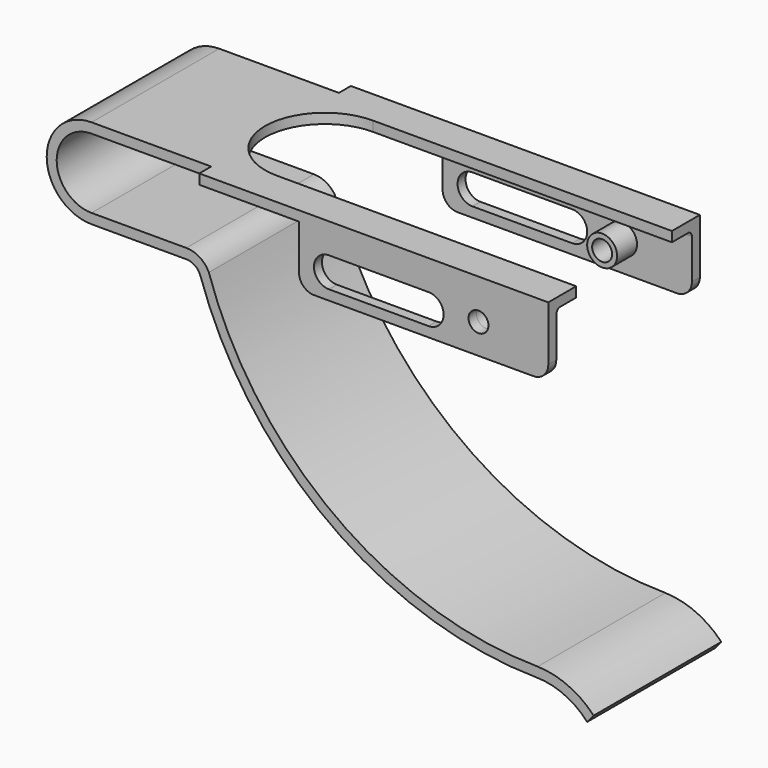
from build123d import *

# Parameters (mm, degrees)
F1_DEPTH  = 16
F2_W      = 70
F2_H      = 3
F3_DEPTH  = 2
F4_W      = 50
F4_H      = 14
F5_DEPTH  = 2
F6_R      = 1
F9_DEPTH  = 2
F11_DEPTH = 38.001
F13_D     = 4
F14_R     = 3
F14_R_2   = 2
F15_DEPTH = 5
F16_R     = 3


# Not quite as in the source:
# - a pattern or mirror of a feature is missing from the dataset's text; its kind, count and spacing are read off the source's solid


with BuildPart() as f1:
    # F0 (on Front) → F1 (new body)
    with BuildSketch(Plane.XZ):
        with BuildLine():
            Line((94, 9), (0, 9))
            ThreePointArc((0, 9), (-9, 0), (0, -9))
            Line((0, -9), (19, -9))
            ThreePointArc((19, -9), (20.7502012229, -9.5634459417), (21.8429732618, -11.0421362138))
            ThreePointArc((21.8429732618, -11.0421362138), (47.7390385011, -46.2740019539), (89.2552166837, -59.996155849))
            ThreePointArc((89.2552166837, -59.996155849), (94.7998907394, -61.2192390349), (99.4028141151, -64.5437599417))
            Line((99.4028141151, -64.5437599417), (100.6981825128, -63))
            ThreePointArc((100.6981825128, -63), (95.5856099225, -59.3797463332), (89.4748869571, -58))
            ThreePointArc((89.4748869571, -58), (48.7477072094, -44.5420257674), (23.5164318764, -9.8548093079))
            ThreePointArc((23.5164318764, -9.8548093079), (21.6715207784, -7.7735385095), (19, -7))
            Line((19, -7), (0, -7))
            ThreePointArc((0, -7), (-7, 0), (0, 7))
            Line((0, 7), (94, 7))
            Line((94, 7), (94, 9))
        make_face()
    extrude(amount=F1_DEPTH)

    # F2 (on face) → F3 (join)
    with BuildSketch(Plane.XY.offset(9)):
        with Locations((59, -17.5)):
            Rectangle(F2_W, F2_H)
    extrude(amount=-F3_DEPTH)

    # F4 (on face) → F5 (join)
    with BuildSketch(Plane.XZ.offset(19)):
        with Locations((69, 2)):
            Rectangle(F4_W, F4_H)
    extrude(amount=-F5_DEPTH)

    # F6
    f6_edges = [f1.edges().sort_by_distance(p)[0] for p in [
        (69, -17, 7),
    ]]
    fillet(f6_edges, radius=F6_R)

    # F7: F1 across plane


with BuildPart() as f1_1:
    add(f1.part)
    add(f1.part.mirror(Plane.XZ))

    # F8 (on face) → F9 (cut)
    with BuildSketch(Plane.XY.offset(9)):
        with BuildLine():
            Line((94, 12), (34, 12))
            ThreePointArc((34, 12), (22, 0), (34, -12))
            Line((34, -12), (94, -12))
            Line((94, -12), (94, 12))
        make_face()
    extrude(amount=-F9_DEPTH, mode=Mode.SUBTRACT)

    # F10 (on face) → F11 (cut, through all)
    with BuildSketch(Plane.XZ.offset(19)):
        with BuildLine():
            ThreePointArc((50, 3), (47, 0), (50, -3))
            Line((50, -3), (70, -3))
            ThreePointArc((70, -3), (73, 0), (70, 3))
            Line((70, 3), (50, 3))
        make_face()
    extrude(amount=-F11_DEPTH, mode=Mode.SUBTRACT)

    # F13 (through all)
    with Locations(Plane.XZ.offset(19)):
        with Locations((80, 1)):
            Hole(F13_D / 2)

    # F14 (on face) → F15 (join)
    with BuildSketch(Plane(origin=(0, -17, 0), x_dir=(-1, 0, 0), z_dir=(0, 1, 0))):
        with Locations((-80, 1)):
            Circle(F14_R)
        with Locations((-80, 1)):
            Circle(F14_R_2, mode=Mode.SUBTRACT)
    f15 = extrude(amount=F15_DEPTH)

    # F15_copies: F15 across plane
    add(f15.mirror(Plane.ZX))

    # F16
    f16_edges = [f1_1.edges().sort_by_distance(p)[0] for p in [
        (94, -18, -5),
        (44, -18, -5),
        (94, 18, -5),
        (44, 18, -5),
    ]]
    fillet(f16_edges, radius=F16_R)


solid = f1_1.part
